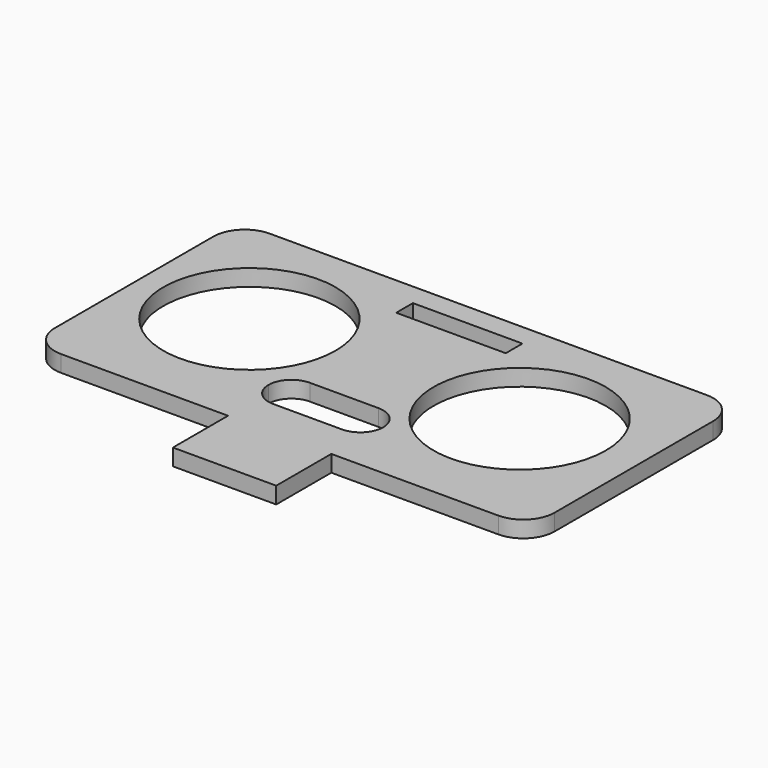
from build123d import *

# Parameters (mm, degrees)
F2_R     = 8.25
F2_W     = 9.9
F2_H     = 6.6
F3_DEPTH = 1.5875
F4_W     = 11
F4_H     = 4.4
F4_W_2   = 10.5
F4_H_2   = 2
F5_DEPTH = 1.5885
F6_R     = 3
F7_R     = 2.19999


# Not quite as in the source:
# - a fillet or chamfer is up to 0.001 mm smaller than in the source, because OpenCascade refuses the exact size


with BuildPart() as f3:
    # F2 (on Top) → F3 (new body)
    with BuildSketch(Plane.XY):
        Polygon((-23.95, 25), (-23.95, 0), (-4.95, 0), (4.95, 0), (23.95, 0), (23.95, 25), align=None)
        with Locations((-13.5, 13.25)):
            Circle(F2_R, mode=Mode.SUBTRACT)
        with Locations((12.4, 13.25)):
            Circle(F2_R, mode=Mode.SUBTRACT)
        with Locations((0, -3.3)):
            Rectangle(F2_W, F2_H)
    extrude(amount=F3_DEPTH)

    # F4 (on face) → F5 (cut, through all)
    with BuildSketch(Plane.XY.offset(1.5875)):
        with Locations((-0.2067205198, 5.8)):
            Rectangle(F4_W, F4_H)
        with Locations((-0.3, 21.9)):
            Rectangle(F4_W_2, F4_H_2)
    extrude(amount=-F5_DEPTH, mode=Mode.SUBTRACT)

    # F6
    f6_edges = [f3.edges().sort_by_distance(p)[0] for p in [
        (-23.95, 0, 0.79375),
        (-23.95, 25, 0.79375),
        (23.95, 25, 0.79375),
        (23.95, 0, 0.79375),
    ]]
    fillet(f6_edges, radius=F6_R)

    # F7 (radius 2.2 in the source; OpenCascade refuses exactly that, so slightly less here)
    f7_edges = [f3.edges().sort_by_distance(p)[0] for p in [
        (-5.706721, 3.6, 0.79375),
        (-5.706721, 8, 0.79375),
        (5.293279, 3.6, 0.79375),
        (5.293279, 8, 0.79375),
    ]]
    fillet(f7_edges, radius=F7_R)


solid = f3.part
